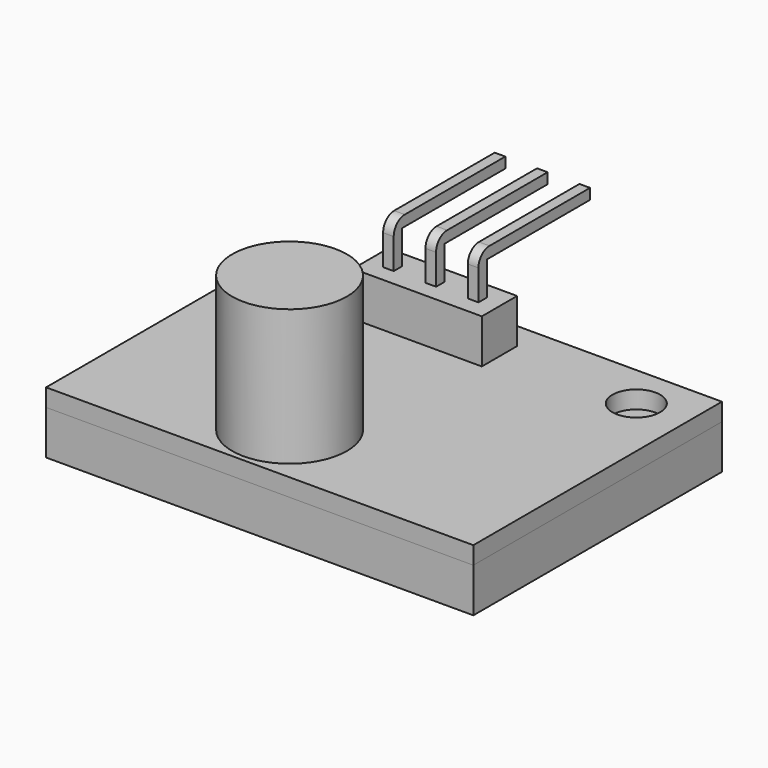
from build123d import *

# Parameters (mm, degrees)
F0_W      = 24.2
F0_H      = 17.6
F0_R      = 1.35
F1_DEPTH  = 1
F2_W      = 7.3
F2_H      = 2.5
F2_W_2    = 0.6
F2_H_2    = 0.6
F3_DEPTH  = 2.5
F4_W      = 0.6
F4_H      = 0.6
F5_DEPTH  = 5
F6_W      = 0.6
F6_H      = 0.6
F7_DEPTH  = 7.5
F8_R      = 0.781625783
F8_2_R    = 0.781625783
F8_3_R    = 0.781625783
F9_SIZE   = 0.2
F9_2_SIZE = 0.2
F9_3_SIZE = 0.2
F10_R     = 3.25
F11_DEPTH = 7.7
F12_W     = 24.2
F12_H     = 17.6
F12_R     = 1.35
F13_DEPTH = 2.5


with BuildPart() as f1:
    # F0 (on Top) → F1 (new body)
    with BuildSketch(Plane.XY):
        with Locations((-0.4637802485, -0.4887992391)):
            Rectangle(F0_W, F0_H)
        with Locations((-9.6137802485, 5.8112007609)):
            Circle(F0_R, mode=Mode.SUBTRACT)
        with Locations((8.7862197515, 5.8112007609)):
            Circle(F0_R, mode=Mode.SUBTRACT)
    extrude(amount=F1_DEPTH)


with BuildPart() as f3:
    # F2 (on face) → F3 (new body)
    with BuildSketch(Plane.XY.offset(1)):
        with Locations((-2.4137802485, 5.5612007609)):
            Rectangle(F2_W, F2_H)
        with Locations((-4.8137802485, 5.5612007609)):
            Rectangle(F2_W_2, F2_H_2, mode=Mode.SUBTRACT)
        with Locations((-2.4137802485, 5.5612007609)):
            Rectangle(F2_W_2, F2_H_2, mode=Mode.SUBTRACT)
        with Locations((-0.0137802485, 5.5612007609)):
            Rectangle(F2_W_2, F2_H_2, mode=Mode.SUBTRACT)
    extrude(amount=F3_DEPTH)


with BuildPart() as f5:
    # F4 (on face) → F5 (new body)
    with BuildSketch(Plane.XY.offset(1)):
        with Locations((-4.8137802485, 5.5612007609)):
            Rectangle(F4_W, F4_H)
    extrude(amount=F5_DEPTH)

    # F6 (on face) → F7, piece 3 (join)
    with BuildSketch(Plane(origin=(0, 5.8612007609, 0), x_dir=(-1, 0, 0), z_dir=(0, 1, 0))):
        with Locations((4.8137802485, 5.7)):
            Rectangle(F6_W, F6_H)
    extrude(amount=F7_DEPTH)

    # F8
    f8_edges = [f5.edges().sort_by_distance(p)[0] for p in [
        (-4.81378, 5.261201, 6),
    ]]
    fillet(f8_edges, radius=F8_R)

    # F9
    f9_edges = [f5.edges().sort_by_distance(p)[0] for p in [
        (-4.81378, 13.361201, 6),
        (-4.51378, 13.361201, 5.7),
        (-4.81378, 13.361201, 5.4),
        (-5.11378, 13.361201, 5.7),
    ]]
    chamfer(f9_edges, length=F9_SIZE)


with BuildPart() as f5b:
    # F4 (on face) → F5, piece 2 (new body)
    with BuildSketch(Plane.XY.offset(1)):
        with Locations((-2.4137802485, 5.5612007609)):
            Rectangle(F4_W, F4_H)
    extrude(amount=F5_DEPTH)

    # F6 (on face) → F7, piece 2 (join)
    with BuildSketch(Plane(origin=(0, 5.8612007609, 0), x_dir=(-1, 0, 0), z_dir=(0, 1, 0))):
        with Locations((2.4137802485, 5.7)):
            Rectangle(F6_W, F6_H)
    extrude(amount=F7_DEPTH)

    # F8#2
    f8_2_edges = [f5b.edges().sort_by_distance(p)[0] for p in [
        (-2.41378, 5.261201, 6),
    ]]
    fillet(f8_2_edges, radius=F8_2_R)

    # F9#2
    f9_2_edges = [f5b.edges().sort_by_distance(p)[0] for p in [
        (-2.11378, 13.361201, 5.7),
        (-2.41378, 13.361201, 6),
        (-2.41378, 13.361201, 5.4),
        (-2.71378, 13.361201, 5.7),
    ]]
    chamfer(f9_2_edges, length=F9_2_SIZE)


with BuildPart() as f5c:
    # F4 (on face) → F5, piece 3 (new body)
    with BuildSketch(Plane.XY.offset(1)):
        with Locations((-0.0137802485, 5.5612007609)):
            Rectangle(F4_W, F4_H)
    extrude(amount=F5_DEPTH)

    # F6 (on face) → F7 (join)
    with BuildSketch(Plane(origin=(0, 5.8612007609, 0), x_dir=(-1, 0, 0), z_dir=(0, 1, 0))):
        with Locations((0.0137802485, 5.7)):
            Rectangle(F6_W, F6_H)
    extrude(amount=F7_DEPTH)

    # F8#3
    f8_3_edges = [f5c.edges().sort_by_distance(p)[0] for p in [
        (-0.01378, 5.261201, 6),
    ]]
    fillet(f8_3_edges, radius=F8_3_R)

    # F9#3
    f9_3_edges = [f5c.edges().sort_by_distance(p)[0] for p in [
        (-0.01378, 13.361201, 6),
        (-0.01378, 13.361201, 5.4),
        (0.28622, 13.361201, 5.7),
        (-0.31378, 13.361201, 5.7),
    ]]
    chamfer(f9_3_edges, length=F9_3_SIZE)


with BuildPart() as f11:
    # F10 (on face) → F11 (new body)
    with BuildSketch(Plane.XY.offset(1)):
        with Locations((-1.6137802485, -5.7387992391)):
            Circle(F10_R)
    extrude(amount=F11_DEPTH)


with BuildPart() as f13:
    # F12 (on face) → F13 (new body)
    with BuildSketch(Plane(origin=(0, 0, 0), x_dir=(1, 0, 0), z_dir=(0, 0, -1))):
        with Locations((-0.4637802485, 0.4887992391)):
            Rectangle(F12_W, F12_H)
        with Locations((-9.6137802485, -5.8112007609)):
            Circle(F12_R, mode=Mode.SUBTRACT)
        with Locations((8.7862197515, -5.8112007609)):
            Circle(F12_R, mode=Mode.SUBTRACT)
        with Locations((-9.6137802485, -5.8112007609)):
            Circle(F12_R)
        with Locations((8.7862197515, -5.8112007609)):
            Circle(F12_R)
    extrude(amount=F13_DEPTH)


solid = Compound([f1.part, f3.part, f5.part, f5b.part, f5c.part, f11.part, f13.part])
